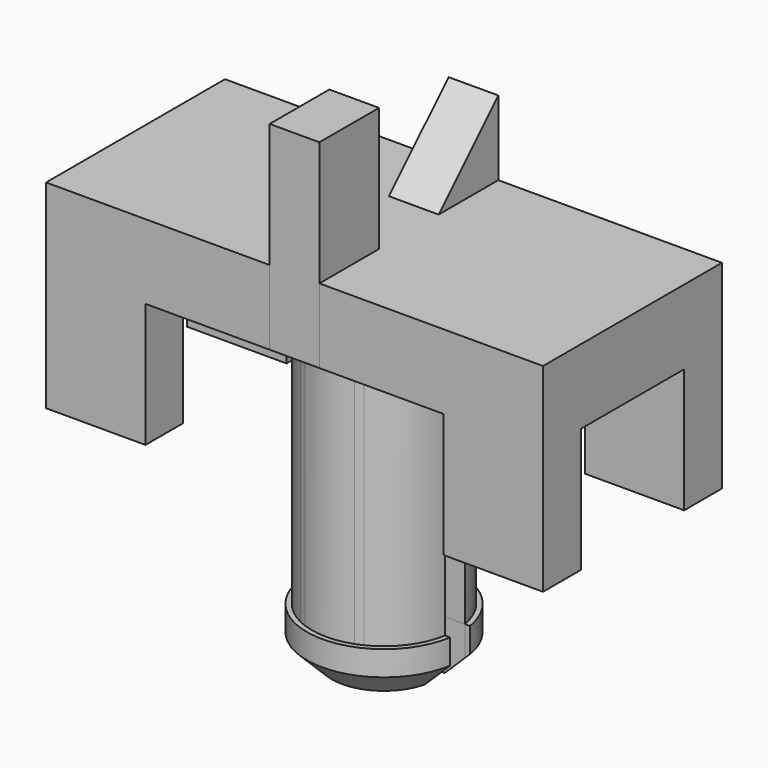
from build123d import *

# Parameters (mm, degrees)
F0_W          = 2
F0_H          = 1.1
F0_H_2        = 1
F1_DEPTH      = 10.5
F2_DEPTH      = 8
F0_W_2        = 4
F0_H_3        = 1.9
F3_DEPTH      = 3
F4_DEPTH      = 5
F5_T1_DEPTH   = 27.7168298797
F7_DEPTH      = 2
F8_T2_ANGLE   = 256.6216565717
F8_2_T2_ANGLE = 256.6216565717


# Not quite as in the source:
# - a fillet or chamfer that OpenCascade refuses, or shapes differently, is made with other operations: its cross-section is extruded or revolved along the edge and cut away or added
# - a pattern or mirror of a feature is missing from the dataset's text; its kind, count and spacing are read off the source's solid


with BuildPart() as f1:
    # F0 (on Top) → F1 (new body)
    with BuildSketch(Plane.XY):
        with BuildLine():
            Line((-2.8565713714, 0.5), (-1, 0.5))
            Line((-1, 0.5), (-1, 1.5))
            Line((-1, 1.5), (-1, 2.6))
            Line((-1, 2.6), (-1.2845232579, 2.6))
            ThreePointArc((-1.2845232579, 2.6), (-2.3215654594, 1.7379107623), (-2.8565713714, 0.5))
        make_face()
        with Locations((0, 2.05)):
            Rectangle(F0_W, F0_H)
        with Locations((0, 1)):
            Rectangle(F0_W, F0_H_2)
        with BuildLine():
            Line((1, 0.5), (2.8565713714, 0.5))
            ThreePointArc((2.8565713714, 0.5), (2.3215654594, 1.7379107623), (1.2845232579, 2.6))
            Line((1.2845232579, 2.6), (1, 2.6))
            Line((1, 2.6), (1, 1.5))
            Line((1, 1.5), (1, 0.5))
        make_face()
        with BuildLine():
            Line((1, 2.6), (1, 2.7221315178))
            ThreePointArc((1, 2.7221315178), (0, 2.9), (-1, 2.7221315178))
            Line((-1, 2.7221315178), (-1, 2.6))
            Line((-1, 2.6), (1, 2.6))
        make_face()
        with BuildLine():
            Line((-1, 2.6), (-1, 2.7221315178))
            ThreePointArc((-1, 2.7221315178), (-1.1438927641, 2.6648657272), (-1.2845232579, 2.6))
            Line((-1.2845232579, 2.6), (-1, 2.6))
        make_face()
        with BuildLine():
            Line((1, 2.6), (1.2845232579, 2.6))
            ThreePointArc((1.2845232579, 2.6), (1.1438927641, 2.6648657272), (1, 2.7221315178))
            Line((1, 2.7221315178), (1, 2.6))
        make_face()
    extrude(amount=-F1_DEPTH)


with BuildPart() as f1b:
    # F0 (on Top) → F1, piece 2 (new body)
    with BuildSketch(Plane.XY):
        with BuildLine():
            ThreePointArc((1.2845232579, -2.6), (2.3215654594, -1.7379107623), (2.8565713714, -0.5))
            Line((2.8565713714, -0.5), (1, -0.5))
            Line((1, -0.5), (1, -1.5))
            Line((1, -1.5), (1, -2.6))
            Line((1, -2.6), (1.2845232579, -2.6))
        make_face()
        with Locations((0, -2.05)):
            Rectangle(F0_W, F0_H)
        with Locations((0, -1)):
            Rectangle(F0_W, F0_H_2)
        with BuildLine():
            Line((-1, -1.5), (-1, -0.5))
            Line((-1, -0.5), (-2.8565713714, -0.5))
            ThreePointArc((-2.8565713714, -0.5), (-2.3215654594, -1.7379107623), (-1.2845232579, -2.6))
            Line((-1.2845232579, -2.6), (-1, -2.6))
            Line((-1, -2.6), (-1, -1.5))
        make_face()
        with BuildLine():
            ThreePointArc((-1, -2.7221315178), (0, -2.9), (1, -2.7221315178))
            Line((1, -2.7221315178), (1, -2.6))
            Line((1, -2.6), (-1, -2.6))
            Line((-1, -2.6), (-1, -2.7221315178))
        make_face()
        with BuildLine():
            ThreePointArc((-1.2845232579, -2.6), (-1.1438927641, -2.6648657272), (-1, -2.7221315178))
            Line((-1, -2.7221315178), (-1, -2.6))
            Line((-1, -2.6), (-1.2845232579, -2.6))
        make_face()
        with BuildLine():
            ThreePointArc((1, -2.7221315178), (1.1438927641, -2.6648657272), (1.2845232579, -2.6))
            Line((1.2845232579, -2.6), (1, -2.6))
            Line((1, -2.6), (1, -2.7221315178))
        make_face()
    extrude(amount=-F1_DEPTH)


with BuildPart() as f2:
    # F0 (on Top) → F2 (new body)
    with BuildSketch(Plane.XY):
        with BuildLine():
            ThreePointArc((-1, 2.7221315178), (0, 2.9), (1, 2.7221315178))
            Line((1, 2.7221315178), (1, 4.5))
            Line((1, 4.5), (-1, 4.5))
            Line((-1, 4.5), (-1, 2.7221315178))
        make_face()
        with Locations((0, 2.05)):
            Rectangle(F0_W, F0_H)
        with BuildLine():
            Line((1, 2.6), (1, 2.7221315178))
            ThreePointArc((1, 2.7221315178), (0, 2.9), (-1, 2.7221315178))
            Line((-1, 2.7221315178), (-1, 2.6))
            Line((-1, 2.6), (1, 2.6))
        make_face()
    extrude(amount=F2_DEPTH)

    # F5: chamfer of 5 on 1 edges, made by hand

    # F5_s2 → F5_t1 (cut)
    with BuildSketch(Plane.YZ.offset(-13.8584149398)):
        Polygon((1.5, 3), (6.5, 8), (1.5, 8), align=None)
    extrude(amount=F5_T1_DEPTH, mode=Mode.SUBTRACT)


with BuildPart() as f2b:
    # F0 (on Top) → F2, piece 2 (new body)
    with BuildSketch(Plane.XY):
        with Locations((0, -2.05)):
            Rectangle(F0_W, F0_H)
        with BuildLine():
            ThreePointArc((-1, -2.7221315178), (0, -2.9), (1, -2.7221315178))
            Line((1, -2.7221315178), (1, -2.6))
            Line((1, -2.6), (-1, -2.6))
            Line((-1, -2.6), (-1, -2.7221315178))
        make_face()
        with BuildLine():
            Line((1, -4.5), (1, -2.7221315178))
            ThreePointArc((1, -2.7221315178), (0, -2.9), (-1, -2.7221315178))
            Line((-1, -2.7221315178), (-1, -4.5))
            Line((-1, -4.5), (1, -4.5))
        make_face()
    extrude(amount=F2_DEPTH)


with BuildPart() as f3:
    # F0 (on Top) → F3 (new body)
    with BuildSketch(Plane.XY):
        with BuildLine():
            ThreePointArc((-1.2845232579, 2.6), (-1.1438927641, 2.6648657272), (-1, 2.7221315178))
            Line((-1, 2.7221315178), (-1, 4.5))
            Line((-1, 4.5), (-6, 4.5))
            Line((-6, 4.5), (-6, 2.6))
            Line((-6, 2.6), (-1.2845232579, 2.6))
        make_face()
        with BuildLine():
            Line((-10, 0.5), (-2.8565713714, 0.5))
            ThreePointArc((-2.8565713714, 0.5), (-2.3215654594, 1.7379107623), (-1.2845232579, 2.6))
            Line((-1.2845232579, 2.6), (-6, 2.6))
            Line((-6, 2.6), (-10, 2.6))
            Line((-10, 2.6), (-10, 0.5))
        make_face()
        with BuildLine():
            Line((-2.8565713714, 0.5), (-1, 0.5))
            Line((-1, 0.5), (-1, 1.5))
            Line((-1, 1.5), (-1, 2.6))
            Line((-1, 2.6), (-1.2845232579, 2.6))
            ThreePointArc((-1.2845232579, 2.6), (-2.3215654594, 1.7379107623), (-2.8565713714, 0.5))
        make_face()
        with BuildLine():
            ThreePointArc((-2.8565713714, -0.5), (-2.9, 0), (-2.8565713714, 0.5))
            Line((-2.8565713714, 0.5), (-10, 0.5))
            Line((-10, 0.5), (-10, -0.5))
            Line((-10, -0.5), (-2.8565713714, -0.5))
        make_face()
        with BuildLine():
            Line((-1, -0.5), (-1, 0.5))
            Line((-1, 0.5), (-2.8565713714, 0.5))
            ThreePointArc((-2.8565713714, 0.5), (-2.9, 0), (-2.8565713714, -0.5))
            Line((-2.8565713714, -0.5), (-1, -0.5))
        make_face()
        with BuildLine():
            Line((-1, -1.5), (-1, -0.5))
            Line((-1, -0.5), (-2.8565713714, -0.5))
            ThreePointArc((-2.8565713714, -0.5), (-2.3215654594, -1.7379107623), (-1.2845232579, -2.6))
            Line((-1.2845232579, -2.6), (-1, -2.6))
            Line((-1, -2.6), (-1, -1.5))
        make_face()
        with BuildLine():
            ThreePointArc((-1.2845232579, -2.6), (-2.3215654594, -1.7379107623), (-2.8565713714, -0.5))
            Line((-2.8565713714, -0.5), (-10, -0.5))
            Line((-10, -0.5), (-10, -2.6))
            Line((-10, -2.6), (-6, -2.6))
            Line((-6, -2.6), (-1.2845232579, -2.6))
        make_face()
        with BuildLine():
            Line((-1, -4.5), (-1, -2.7221315178))
            ThreePointArc((-1, -2.7221315178), (-1.1438927641, -2.6648657272), (-1.2845232579, -2.6))
            Line((-1.2845232579, -2.6), (-6, -2.6))
            Line((-6, -2.6), (-6, -4.5))
            Line((-6, -4.5), (-1, -4.5))
        make_face()
        with Locations((0, 1)):
            Rectangle(F0_W, F0_H_2)
        Rectangle(F0_W, F0_H_2)
        with Locations((0, -1)):
            Rectangle(F0_W, F0_H_2)
        with BuildLine():
            ThreePointArc((1, 2.7221315178), (1.1438927641, 2.6648657272), (1.2845232579, 2.6))
            Line((1.2845232579, 2.6), (6, 2.6))
            Line((6, 2.6), (6, 4.5))
            Line((6, 4.5), (1, 4.5))
            Line((1, 4.5), (1, 2.7221315178))
        make_face()
        with BuildLine():
            Line((1, 0.5), (2.8565713714, 0.5))
            ThreePointArc((2.8565713714, 0.5), (2.3215654594, 1.7379107623), (1.2845232579, 2.6))
            Line((1.2845232579, 2.6), (1, 2.6))
            Line((1, 2.6), (1, 1.5))
            Line((1, 1.5), (1, 0.5))
        make_face()
        with BuildLine():
            Line((1, 2.6), (1.2845232579, 2.6))
            ThreePointArc((1.2845232579, 2.6), (1.1438927641, 2.6648657272), (1, 2.7221315178))
            Line((1, 2.7221315178), (1, 2.6))
        make_face()
        with BuildLine():
            ThreePointArc((1.2845232579, 2.6), (2.3215654594, 1.7379107623), (2.8565713714, 0.5))
            Line((2.8565713714, 0.5), (10, 0.5))
            Line((10, 0.5), (10, 2.6))
            Line((10, 2.6), (6, 2.6))
            Line((6, 2.6), (1.2845232579, 2.6))
        make_face()
        with BuildLine():
            ThreePointArc((2.8565713714, 0.5), (2.8891224426, 0.250941251), (2.9, 0))
            ThreePointArc((2.9, 0), (2.8891224426, -0.250941251), (2.8565713714, -0.5))
            Line((2.8565713714, -0.5), (10, -0.5))
            Line((10, -0.5), (10, 0.5))
            Line((10, 0.5), (2.8565713714, 0.5))
        make_face()
        with BuildLine():
            ThreePointArc((2.8565713714, -0.5), (2.8891224426, -0.250941251), (2.9, 0))
            ThreePointArc((2.9, 0), (2.8891224426, 0.250941251), (2.8565713714, 0.5))
            Line((2.8565713714, 0.5), (1, 0.5))
            Line((1, 0.5), (1, -0.5))
            Line((1, -0.5), (2.8565713714, -0.5))
        make_face()
        with BuildLine():
            ThreePointArc((1.2845232579, -2.6), (2.3215654594, -1.7379107623), (2.8565713714, -0.5))
            Line((2.8565713714, -0.5), (1, -0.5))
            Line((1, -0.5), (1, -1.5))
            Line((1, -1.5), (1, -2.6))
            Line((1, -2.6), (1.2845232579, -2.6))
        make_face()
        with BuildLine():
            Line((10, -0.5), (2.8565713714, -0.5))
            ThreePointArc((2.8565713714, -0.5), (2.3215654594, -1.7379107623), (1.2845232579, -2.6))
            Line((1.2845232579, -2.6), (6, -2.6))
            Line((6, -2.6), (10, -2.6))
            Line((10, -2.6), (10, -0.5))
        make_face()
        with BuildLine():
            ThreePointArc((1, -2.7221315178), (1.1438927641, -2.6648657272), (1.2845232579, -2.6))
            Line((1.2845232579, -2.6), (1, -2.6))
            Line((1, -2.6), (1, -2.7221315178))
        make_face()
        with BuildLine():
            Line((6, -2.6), (1.2845232579, -2.6))
            ThreePointArc((1.2845232579, -2.6), (1.1438927641, -2.6648657272), (1, -2.7221315178))
            Line((1, -2.7221315178), (1, -4.5))
            Line((1, -4.5), (6, -4.5))
            Line((6, -4.5), (6, -2.6))
        make_face()
        with BuildLine():
            ThreePointArc((-1.2845232579, -2.6), (-1.1438927641, -2.6648657272), (-1, -2.7221315178))
            Line((-1, -2.7221315178), (-1, -2.6))
            Line((-1, -2.6), (-1.2845232579, -2.6))
        make_face()
        with BuildLine():
            Line((-1, 2.6), (-1, 2.7221315178))
            ThreePointArc((-1, 2.7221315178), (-1.1438927641, 2.6648657272), (-1.2845232579, 2.6))
            Line((-1.2845232579, 2.6), (-1, 2.6))
        make_face()
        with Locations((-8, 3.55)):
            Rectangle(F0_W_2, F0_H_3)
        with Locations((-8, -3.55)):
            Rectangle(F0_W_2, F0_H_3)
        with Locations((8, 3.55)):
            Rectangle(F0_W_2, F0_H_3)
        with Locations((8, -3.55)):
            Rectangle(F0_W_2, F0_H_3)
    extrude(amount=F3_DEPTH)

    # F0 (on Top) → F4 (join)
    with BuildSketch(Plane.XY):
        with Locations((-8, -3.55)):
            Rectangle(F0_W_2, F0_H_3)
        with Locations((-8, 3.55)):
            Rectangle(F0_W_2, F0_H_3)
        with Locations((8, -3.55)):
            Rectangle(F0_W_2, F0_H_3)
        with Locations((8, 3.55)):
            Rectangle(F0_W_2, F0_H_3)
    extrude(amount=-F4_DEPTH)


with BuildPart() as f7:
    # F6 (on face) → F7 (new body)
    with BuildSketch(Plane(origin=(0, 0, -10.5), x_dir=(1, 0, 0), z_dir=(0, 0, -1))):
        with BuildLine():
            Line((0, 0.5), (3.0594117082, 0.5))
            ThreePointArc((3.0594117082, 0.5), (0, 3.1), (-3.0594117082, 0.5))
            Line((-3.0594117082, 0.5), (0, 0.5))
        make_face()
    extrude(amount=F7_DEPTH)


with BuildPart() as f7b:
    # F6 (on face) → F7, piece 2 (new body)
    with BuildSketch(Plane(origin=(0, 0, -10.5), x_dir=(1, 0, 0), z_dir=(0, 0, -1))):
        with BuildLine():
            ThreePointArc((-3.0594117082, -0.5), (0, -3.1), (3.0594117082, -0.5))
            Line((3.0594117082, -0.5), (2.8565713714, -0.5))
            ThreePointArc((2.8565713714, -0.5), (0, -2.9), (-2.8565713714, -0.5))
            Line((-2.8565713714, -0.5), (-3.0594117082, -0.5))
        make_face()
    extrude(amount=F7_DEPTH)

    # F7_copies: F7 across plane
    add(f7.part.mirror(Plane(origin=(0, 4.9e-05, 0), x_dir=(0, 4e-06, 1), z_dir=(0, 1, -4e-06))))

    # F8#2: chamfer of 1 on 2 edges, made by hand

    # F8_2_s1 → F8_2_t2 (revolve, cut)
    with BuildSketch(Plane(origin=(4.76703e-05, 6.03376e-05, -5e-10), x_dir=(0.7846592249, -0.619927335, 0), z_dir=(-0.619927335, -0.7846592249, 6.2773e-06))):
        with BuildLine():
            Line((3.1282804114, -11.471700214), (2.0717171089, -12.5282739965))
            Line((2.0717171089, -12.5282739965), (2.071717208, -12.5482739965))
            ThreePointArc((2.071717208, -12.5482739965), (2.5858592034, -12.5199871754), (3.100001339, -12.5199846256))
            Line((3.100001339, -12.5199846256), (3.1200012398, -12.4999845264))
            ThreePointArc((3.1200012398, -12.4999845264), (3.11999869, -11.9858423908), (3.1482804114, -11.4717001149))
            Line((3.1482804114, -11.4717001149), (3.1282804114, -11.471700214))
        make_face()
    revolve(axis=Axis((0, -2e-06, -12.5), (0, 8e-06, 1)), revolution_arc=F8_2_T2_ANGLE, mode=Mode.SUBTRACT)


with BuildPart() as f7_1:
    add(f7.part)

    # F8: chamfer of 1 on 1 edges, made by hand

    # F8_s1 → F8_t2 (revolve, cut)
    with BuildSketch(Plane(origin=(0, 0, 0), x_dir=(0, 0, 1), z_dir=(-0.619927335, 0.784659225, 0))):
        Polygon((-12.5, 2.1), (-11.5, 3.1), (-12.5, 3.1), align=None)
    revolve(axis=Axis((0, 0, -12.5), (0, 0, -1)), revolution_arc=F8_T2_ANGLE, mode=Mode.SUBTRACT)


solid = Compound([f1.part, f1b.part, f2.part, f2b.part, f3.part, f7b.part, f7_1.part])
